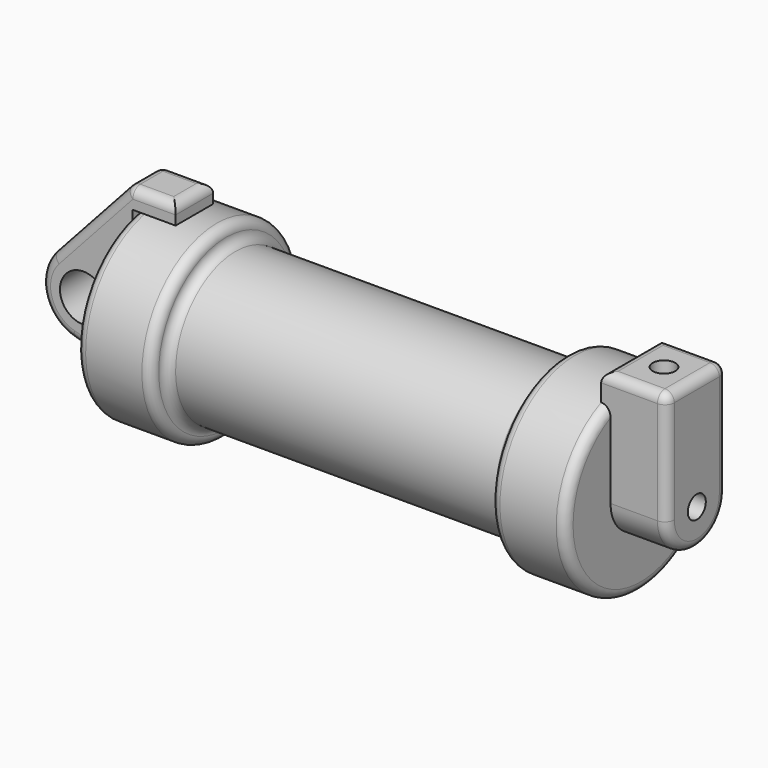
from build123d import *

# Parameters (mm, degrees)
F0_W          = 5.842
F0_H          = 12.7
F2_R          = 1.524
F3_DEPTH      = 7.62
F3_DEPTH_BACK = 1.27
F4_R          = 1.524
F5_DEPTH      = 17.78
F0_R          = 3.175
F6_DEPTH      = 3.175
F7_R          = 1.27
F8_R          = 1.27
F9_R          = 1.26999


# Not quite as in the source:
# - a fillet or chamfer is up to 0.001 mm smaller than in the source, because OpenCascade refuses the exact size


with BuildPart() as f1:
    # F0 (on Front) → F1 (revolve)
    with BuildSketch(Plane.XZ):
        with Locations((2.921, 6.35)):
            Rectangle(F0_W, F0_H)
        Polygon((5.842, 12.7), (5.842, 0), (66.294, 0), (66.294, 12.7), (56.134, 12.7), (56.134, 10.16), (10.16, 10.16), (10.16, 12.7), align=None)
    revolve(axis=Axis((33.147, 0, 0), (-1, 0, 0)))

    # F2 (on face) → F3 (join, two sides)
    with BuildSketch(Plane.YZ.offset(66.294)) as f3_sk:
        with BuildLine():
            ThreePointArc((-5.08, 11.6397422652), (0, 12.7), (5.08, 11.6397422652))
            Line((5.08, 11.6397422652), (5.08, 15.24))
            Line((5.08, 15.24), (-5.08, 15.24))
            Line((-5.08, 15.24), (-5.08, 11.6397422652))
        make_face()
        with BuildLine():
            ThreePointArc((-5.08, 0), (0, 5.08), (5.08, 0))
            Line((5.08, 0), (5.08, 11.6397422652))
            ThreePointArc((5.08, 11.6397422652), (0, 12.7), (-5.08, 11.6397422652))
            Line((-5.08, 11.6397422652), (-5.08, 0))
        make_face()
        with BuildLine():
            ThreePointArc((-5.08, 0), (0, -5.08), (5.08, 0))
            ThreePointArc((5.08, 0), (0, 5.08), (-5.08, 0))
        make_face()
        Circle(F2_R, mode=Mode.SUBTRACT)
    extrude(amount=F3_DEPTH)
    extrude(f3_sk.sketch, amount=-F3_DEPTH_BACK)

    # F4 (on face) → F5 (cut)
    with BuildSketch(Plane.XY.offset(15.24)):
        with Locations((69.469, 0)):
            Circle(F4_R)
    extrude(amount=-F5_DEPTH, mode=Mode.SUBTRACT)

    # F7
    f7_edges = [f1.edges().sort_by_distance(p)[0] for p in [
        (56.134, 0, -10.16),
        (10.16, 0, -10.16),
        (33.147, 0, 10.16),
    ]]
    fillet(f7_edges, radius=F7_R)

    # F9 (radius 1.27 in the source; OpenCascade refuses exactly that, so slightly less here)
    f9_edges = [f1.edges().sort_by_distance(p)[0] for p in [
        (56.134, 0, -12.7),
        (10.16, 0, -12.7),
        (0, 0, -12.7),
        (5.08, 0, 12.7),
        (66.294, 0, -12.7),
        (73.914, 5.08, 7.62),
        (69.469, 5.08, 15.24),
        (69.469, -5.08, 15.24),
        (73.914, 0, 15.24),
        (65.024, 0, 15.24),
    ]]
    fillet(f9_edges, radius=F9_R)


with BuildPart() as f6:
    # F0 (on Front) → F6 (new body, symmetric)
    with BuildSketch(Plane.XZ):
        with BuildLine():
            Line((-0.9398, 0), (0, 0))
            Line((0, 0), (0, 12.7))
            Line((0, 12.7), (5.842, 12.7))
            Line((5.842, 12.7), (5.842, 15.24))
            Line((5.842, 15.24), (-0.508, 15.24))
            Line((-0.508, 15.24), (-10.8806298187, 3.8475430269))
            ThreePointArc((-10.8806298187, 3.8475430269), (-4.5919612295, 5.3297205562), (-0.9398, 0))
        make_face()
        with BuildLine():
            ThreePointArc((-8.1826630726, -5.5069827884), (-3.1957909266, -4.5493385486), (-0.9398, 0))
            ThreePointArc((-0.9398, 0), (-4.5919612295, 5.3297205562), (-10.8806298187, 3.8475430269))
            ThreePointArc((-10.8806298187, 3.8475430269), (-12.1459778134, -1.5837270034), (-8.1826630726, -5.5069827884))
        make_face()
        with Locations((-6.6548, 0)):
            Circle(F0_R, mode=Mode.SUBTRACT)
        with BuildLine():
            Line((5.842, 0), (0, 0))
            Line((0, 0), (-0.9398, 0))
            ThreePointArc((-0.9398, 0), (-3.1957909266, -4.5493385486), (-8.1826630726, -5.5069827884))
            Line((-8.1826630726, -5.5069827884), (5.842, -9.398))
            Line((5.842, -9.398), (5.842, 0))
        make_face()
    extrude(amount=F6_DEPTH, both=True)

    # F8
    f8_edges = [f6.edges().sort_by_distance(p)[0] for p in [
        (5.842, 0, 15.24),
        (2.667, 3.175, 15.24),
        (-0.508, 0, 15.24),
        (2.667, -3.175, 15.24),
        (-5.694315, 3.175, 9.543772),
        (-12.145978, 3.175, -1.583727),
        (-1.170332, 3.175, -7.452491),
        (-1.170332, -3.175, -7.452491),
        (-10.88063, 0, 3.847543),
        (-8.182663, 0, -5.506983),
        (-12.145978, -3.175, -1.583727),
        (-5.694315, -3.175, 9.543772),
    ]]
    fillet(f8_edges, radius=F8_R)


solid = Compound([f1.part, f6.part])
